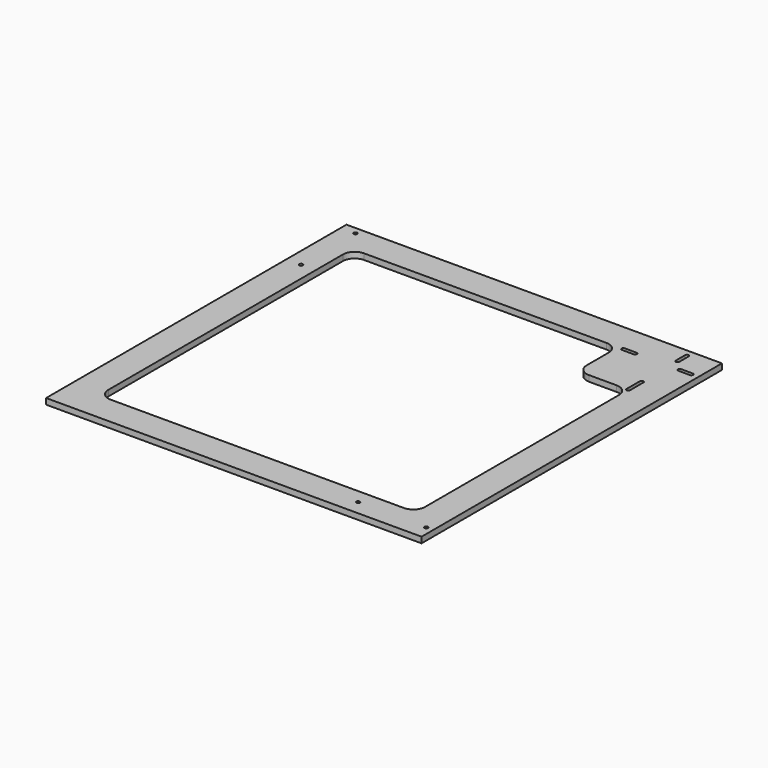
from build123d import *

# Parameters (mm, degrees)
F0_R     = 1.5
F1_DEPTH = 5


# Not quite as in the source:
# - ends of sketch curves that miss each other by under 0.0002 mm in the source are joined


with BuildPart() as f1:
    # F0 (on Top) → F1 (new body)
    with BuildSketch(Plane.XY):
        Polygon((-160, -160), (160, -160), (160, 110), (160, 160), (110, 160), (-160, 160), align=None)
        with Locations((96, -147.5)):
            Circle(F0_R, mode=Mode.SUBTRACT)
        with Locations((154, -147.5)):
            Circle(F0_R, mode=Mode.SUBTRACT)
        with Locations((-147.5, 96)):
            Circle(F0_R, mode=Mode.SUBTRACT)
        with Locations((-147.5, 154)):
            Circle(F0_R, mode=Mode.SUBTRACT)
        with BuildLine():
            ThreePointArc((135, -125), (132.0710678119, -132.0710678119), (125, -135))
            Line((125, -135), (-125, -135))
            ThreePointArc((-125, -135), (-132.0710678119, -132.0710678119), (-135, -125))
            Line((-135, -125), (-135, 125))
            ThreePointArc((-135, 125), (-132.0710678119, 132.0710678119), (-125, 135))
            Line((-125, 135), (81.5, 135))
            ThreePointArc((81.5, 135), (88.5710678119, 132.0710678119), (91.5, 125))
            Line((91.5, 125), (91.5, 101.5))
            ThreePointArc((91.5, 101.5), (94.4289321881, 94.4289321881), (101.5, 91.5))
            Line((101.5, 91.5), (125, 91.5))
            ThreePointArc((125, 91.5), (132.0710678119, 88.5710678119), (135, 81.5))
            Line((135, 81.5), (135, -125))
        make_face(mode=Mode.SUBTRACT)
        with BuildLine():
            ThreePointArc((133.4512195122, 105.877928352), (134.9512195122, 107.377928352), (136.4512195122, 105.877928352))
            Line((136.4512195122, 105.877928352), (136.499991364, 91.5050899728))
            ThreePointArc((136.499991364, 91.5050899728), (135.0025449901, 90.000002159), (133.5, 91.5))
            Line((133.5, 91.5), (133.451236778, 105.8728393094))
            ThreePointArc((133.451236778, 105.8728393094), (133.4512216704, 105.8753838124), (133.4512195122, 105.877928352))
        make_face(mode=Mode.SUBTRACT)
        with BuildLine():
            ThreePointArc((96, 133.5), (94.5, 135), (96, 136.5))
            Line((96, 136.5), (106, 136.5))
            ThreePointArc((106, 136.5), (107.5, 135), (106, 133.5))
            Line((106, 133.5), (96, 133.5))
        make_face(mode=Mode.SUBTRACT)
        with BuildLine():
            ThreePointArc((144, 133.5), (142.5, 135), (144, 136.5))
            Line((144, 136.5), (154, 136.5))
            ThreePointArc((154, 136.5), (155.5, 135), (154, 133.5))
            Line((154, 133.5), (144, 133.5))
        make_face(mode=Mode.SUBTRACT)
        with BuildLine():
            ThreePointArc((133.5, 154), (135, 155.5), (136.5, 154))
            Line((136.5, 154), (136.5, 144))
            ThreePointArc((136.5, 144), (135, 142.5), (133.5, 144))
            Line((133.5, 144), (133.5, 154))
        make_face(mode=Mode.SUBTRACT)
    extrude(amount=F1_DEPTH)


solid = f1.part
